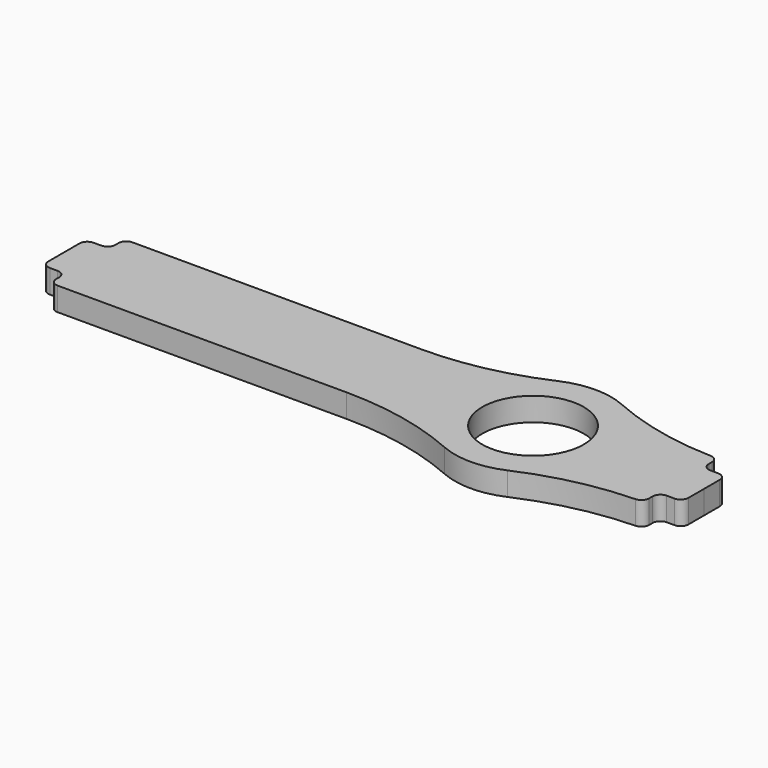
from build123d import *

# Parameters (mm, degrees)
F0_R     = 3.25
F1_DEPTH = 1.5


# Not quite as in the source:
# - ends of sketch curves that miss each other by under 0.0002 mm in the source are joined


with BuildPart() as f1:
    # F0 (on Top) → F1 (new body)
    with BuildSketch(Plane.XY):
        with BuildLine():
            ThreePointArc((11.5751507446, -4.5713014237), (14.9674174979, -3.4491015551), (18.5129609838, -3.00646439))
            ThreePointArc((18.5129609838, -3.00646439), (18.8578988072, -2.8554676082), (18.999681, -2.506641))
            Line((18.999681, -2.506641), (18.999681, -2.236416))
            ThreePointArc((18.999681, -2.236416), (19.1460678639, -1.882922365), (19.499512, -1.7364160286))
            Line((19.499512, -1.7364160286), (19.999851, -1.736246))
            ThreePointArc((19.999851, -1.736246), (20.3532944896, -1.5897392814), (20.499681, -1.236246))
            Line((20.499681, -1.236246), (20.499681, 0.013923))
            Line((20.499681, 0.013923), (20.499257, 1.263923))
            ThreePointArc((20.499257, 1.263923), (20.352690162, 1.6174265783), (19.999087, 1.7637529711))
            Line((19.999087, 1.7637529711), (19.499851, 1.763584))
            ThreePointArc((19.499851, 1.763584), (19.1461877186, 1.9099705104), (18.999681, 2.263584))
            Line((18.999681, 2.263584), (18.999681, 2.50664))
            ThreePointArc((18.999681, 2.50664), (18.8578988072, 2.8554666082), (18.5129609897, 3.0064636108))
            ThreePointArc((18.5129609897, 3.0064636108), (14.9674177085, 3.4491015077), (11.575151115, 4.5713012596))
            ThreePointArc((11.575151115, 4.5713012596), (9.5454328003, 4.9999983336), (7.5164170751, 4.5679878314))
            ThreePointArc((7.5164170751, 4.5679878314), (3.8419543275, 3.3757683124), (-0.000319, 2.9757689864))
            Line((-0.000319, 2.9757689864), (-18.499681, 2.999361))
            ThreePointArc((-18.499681, 2.999361), (-18.4999199994, 2.9993618408), (-18.5001589997, 2.9993619744))
            ThreePointArc((-18.5001589997, 2.9993619744), (-18.853403349, 2.8527463514), (-18.999681, 2.499362))
            Line((-18.999681, 2.499362), (-18.999681, 2.250339))
            ThreePointArc((-18.999681, 2.250339), (-19.1460675104, 1.8968457186), (-19.499511, 1.7503390289))
            Line((-19.499511, 1.7503390289), (-19.999851, 1.75017))
            ThreePointArc((-19.999851, 1.75017), (-20.3532944896, 1.6036632814), (-20.499681, 1.25017))
            Line((-20.499681, 1.25017), (-20.499681, 0))
            Line((-20.499681, 0), (-20.499256, -1.25))
            ThreePointArc((-20.499256, -1.25), (-20.3526895157, -1.6035032249), (-19.999087, -1.7498299714))
            Line((-19.999087, -1.7498299714), (-19.499851, -1.749661))
            ThreePointArc((-19.499851, -1.749661), (-19.1461877186, -1.8960475104), (-18.999681, -2.249661))
            Line((-18.999681, -2.249661), (-18.999681, -2.5))
            ThreePointArc((-18.999681, -2.5), (-18.8532343906, -2.8535533906), (-18.499681, -3))
            Line((-18.499681, -3), (-0.000319, -3))
            ThreePointArc((-0.000319, -3), (3.8532843758, -3.3991955476), (7.5432329323, -4.5798291546))
            ThreePointArc((7.5432329323, -4.5798291546), (9.5600895804, -4.9999888178), (11.5751507446, -4.5713014237))
        make_face()
        with Locations((9.549515, 0)):
            Circle(F0_R, mode=Mode.SUBTRACT)
    extrude(amount=F1_DEPTH)


solid = f1.part
